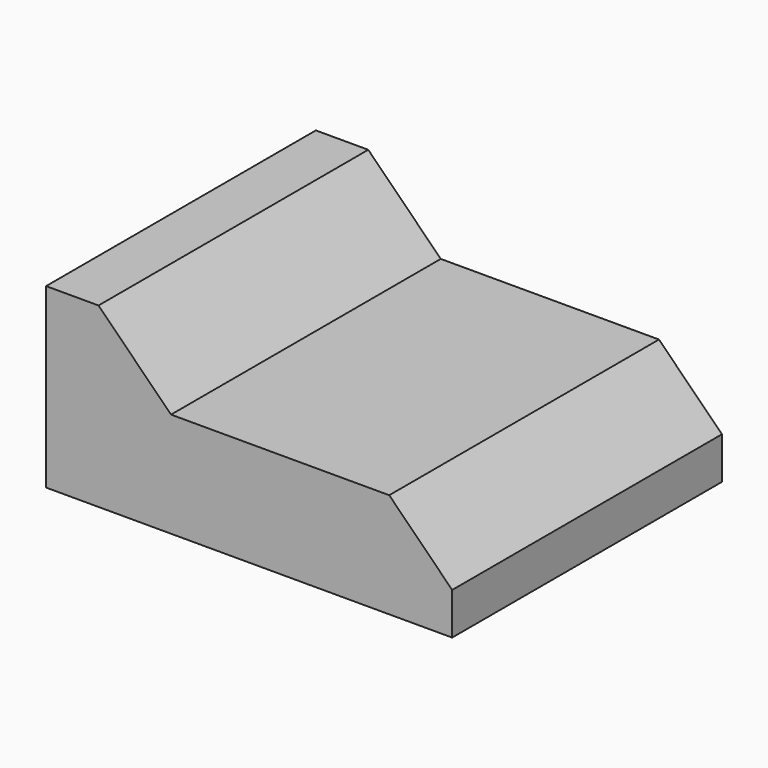
from build123d import *

# Parameters (mm, degrees)
F0_W        = 15.3297632933
F0_H        = 43.554501608
F0_W_2      = 41.3750298321
F0_W_3      = 28.9361141622
F1_DEPTH    = 25.4
F2_W        = 17.5558461342
F2_H        = 43.554501608
F3_DEPTH    = 25.4
F4_SIZE     = 15.24
F5_T4_DEPTH = 174.1959973967
F6_DEPTH    = 12.7
F7_DEPTH    = 25.4
F8_DEPTH    = 12.7


# Not quite as in the source:
# - a fillet or chamfer that OpenCascade refuses, or shapes differently, is made with other operations: its cross-section is extruded or revolved along the edge and cut away or added


with BuildPart() as f1:
    # F0 (on Top) → F1 (new body)
    with BuildSketch(Plane.XY):
        with Locations((-7.6648816466, -1.5181871131)):
            Rectangle(F0_W, F0_H)
        with Locations((20.6875149161, -1.5181871131)):
            Rectangle(F0_W_2, F0_H)
        with Locations((55.8430869132, -1.5181871131)):
            Rectangle(F0_W_3, F0_H)
    extrude(amount=F1_DEPTH)

    # F2 (on face) → F3 (join)
    with BuildSketch(Plane.XY.offset(25.4)):
        with Locations((-6.5518402262, -1.5181871131)):
            Rectangle(F2_W, F2_H)
    extrude(amount=F3_DEPTH)

    # F4
    f4_edges = [f1.edges().sort_by_distance(p)[0] for p in [
        (70.311144, -1.518187, 25.4),
    ]]
    chamfer(f4_edges, length=F4_SIZE)

    # F5: chamfer of 25.4 on 1 edges, made by hand


with BuildPart() as f5_tool2:
    # F5_s3 → F5_t4 (new body)
    with BuildSketch(Plane.XZ.offset(88.6161858114)):
        Polygon((2.2260828409, 25.4), (-23.1739171591, 50.8), (2.2260828409, 50.8), align=None)
    extrude(amount=-F5_T4_DEPTH)

    split(bisect_by=Plane.XY.offset(25.4), keep=Keep.TOP)


with BuildPart() as f1_1:
    add(f1.part)

    # F5_t1: cut F5_tool2
    add(f5_tool2.part, mode=Mode.SUBTRACT)

    # F6 (add): a face of the model
    f6_faces = [f1_1.faces().sort_by_distance(p)[0] for p in [
        (-15.3297632933, -1.5181871131, 21.4779230671),
    ]]
    extrude(f6_faces, amount=F6_DEPTH)

    # F7 (add): a face of the model
    f7_faces = [f1_1.faces().sort_by_distance(p)[0] for p in [
        (14.1137713258, 20.2590636909, 15.1513351417),
    ]]
    extrude(f7_faces, amount=F7_DEPTH)

    # F8 (add): a face of the model
    f8_faces = [f1_1.faces().sort_by_distance(p)[0] for p in [
        (14.1137713258, 45.6590636909, 15.1513351417),
    ]]
    extrude(f8_faces, amount=F8_DEPTH)


solid = f1_1.part
